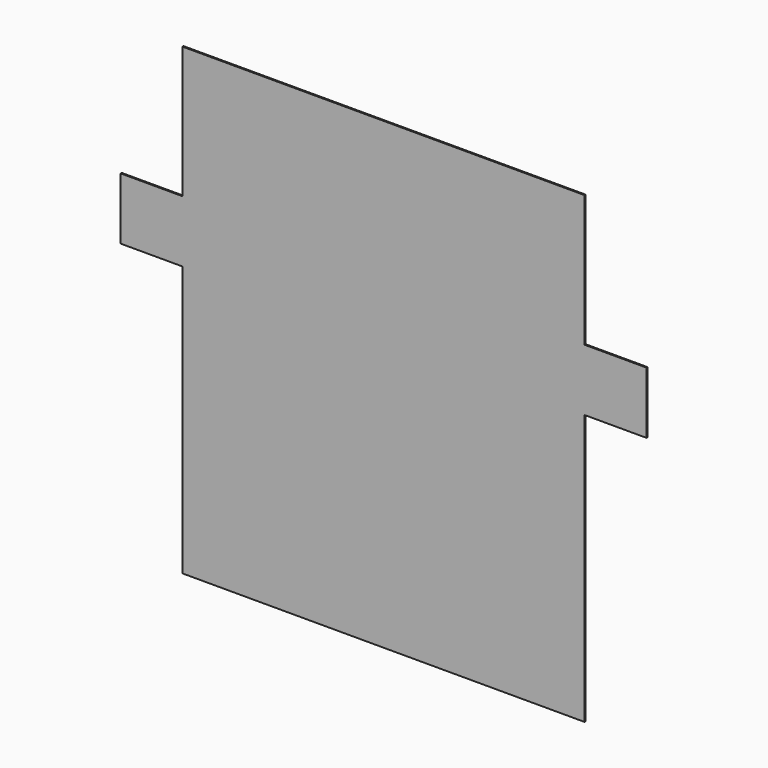
from build123d import *

# Parameters (mm, degrees)
F1_DEPTH = 4


# Not quite as in the source:
# - a feature names something its author has since deleted; it is built from what else it names


with BuildPart() as f1:
    # F0 (on Front) → F1 (new body)
    with BuildSketch(Plane.XZ):
        Polygon((649.293166399, 438.9045192336), (649.293166399, 638.9045192336), (449.293166399, 638.9045192336), (449.293166399, 1064.9045192336), (-850.706833601, 1064.9045192336), (-850.706833601, 638.9045192336), (-1050.706833601, 638.9045192336), (-1050.706833601, 438.9045192336), (-850.706833601, 438.9045192336), (-850.706833601, -435.0954807664), (449.293166399, -435.0954807664), (449.293166399, 438.9045192336), align=None)
    extrude(amount=F1_DEPTH)


solid = f1.part
